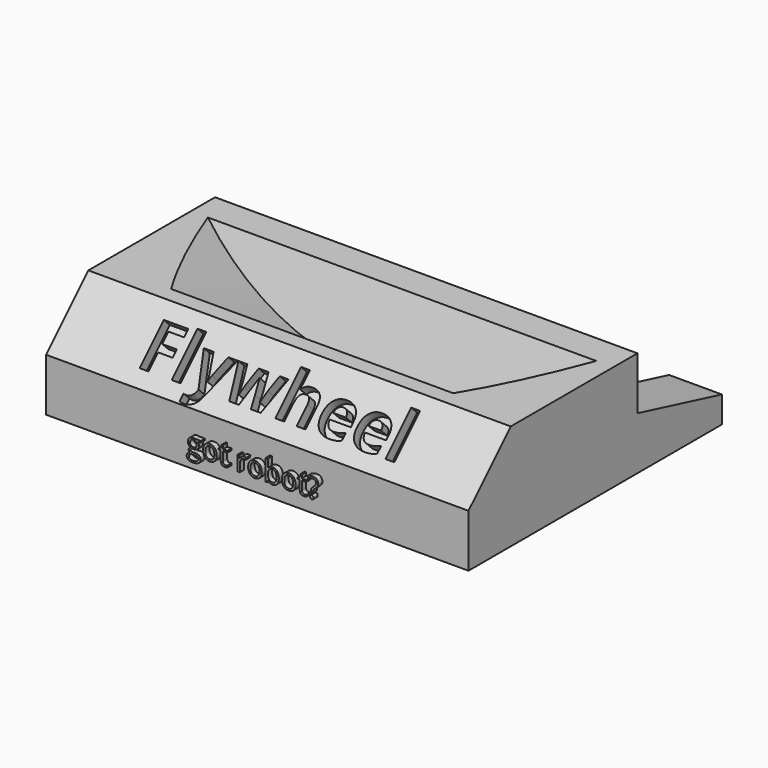
from build123d import *

# Parameters (mm, degrees)
F0_W          = 101.6
F0_H          = 25.4
F1_DEPTH      = 25.4
F4_SIZE       = 12.7
F6_DEPTH      = 101.6
F0_W_2        = 76.2
F7_DEPTH      = 25.4
F8_TEXT_SIZE  = 14.4006236491
F9_DEPTH      = 2.54
F10_TEXT_SIZE = 6.6833958651
F11_DEPTH     = 1.27


# Not quite as in the source:
# - Text() gives the source's letters only with a copy of the font that has no kerning and outlines rounded to 1/6400 em; it was checked with that copy


with BuildPart() as f1:
    # F0 (on Top) → F1 (new body)
    with BuildSketch(Plane.XY):
        with Locations((0, -12.7)):
            Rectangle(F0_W, F0_H)
        Polygon((-38.1, 25.4), (-50.8, 25.4), (-50.8, 0), (50.8, 0), (50.8, 25.4), (38.1, 25.4), align=None)
    extrude(amount=F1_DEPTH)

    # F2 (on Right) → F3 (revolve, cut)
    with BuildSketch(Plane.YZ):
        Polygon((-11.934096284, 17.0436558202), (0, 12.7), (23.6729242203, 77.7408247477), (11.7388279363, 82.0844805679), align=None)
        Polygon((23.6729242203, 77.7408247477), (0, 12.7), (11.934096284, 8.3563441798), (35.6070205043, 73.3971689275), align=None)
    revolve(axis=Axis((0, 29.6399723623, 75.5689968376), (0, 0.9396926208, -0.3420201433)), mode=Mode.SUBTRACT)

    # F4
    f4_edges = [f1.edges().sort_by_distance(p)[0] for p in [
        (0, -25.4, 25.4),
    ]]
    chamfer(f4_edges, length=F4_SIZE)

    # F5 (on face) → F6 (join, through all)
    with BuildSketch(Plane(origin=(-50.8, 0, 0), x_dir=(0, -1, 0), z_dir=(-1, 0, 0))):
        Polygon((-50.8, 0), (-25.4, 0), (-25.4, 12.7), (-50.8, 6.35), align=None)
    extrude(amount=-F6_DEPTH)

    # F0 (on Top) → F7 (cut)
    with BuildSketch(Plane.XY):
        with Locations((0, 38.1)):
            Rectangle(F0_W_2, F0_H)
    extrude(amount=F7_DEPTH, mode=Mode.SUBTRACT)

    # F8 (on face) → F9 (cut)
    with BuildSketch(Plane(origin=(0, -19.05, 19.05), x_dir=(1, 0, 0), z_dir=(0, -0.7071067812, 0.7071067812))):
        with Locations((-31.75, -5.1868490273)):
            Text('Flywheel', F8_TEXT_SIZE, font='Open Sans', font_style=FontStyle.BOLD, text_align=(TextAlign.LEFT, TextAlign.BOTTOM))
    extrude(amount=-F9_DEPTH, mode=Mode.SUBTRACT)

    # F10 (on face) → F11 (join)
    with BuildSketch(Plane.XZ.offset(25.4)):
        with Locations((-16.0887091242, 3.81)):
            Text('got robot?', F10_TEXT_SIZE, font='Open Sans', text_align=(TextAlign.LEFT, TextAlign.BOTTOM))
    extrude(amount=F11_DEPTH)


solid = f1.part
